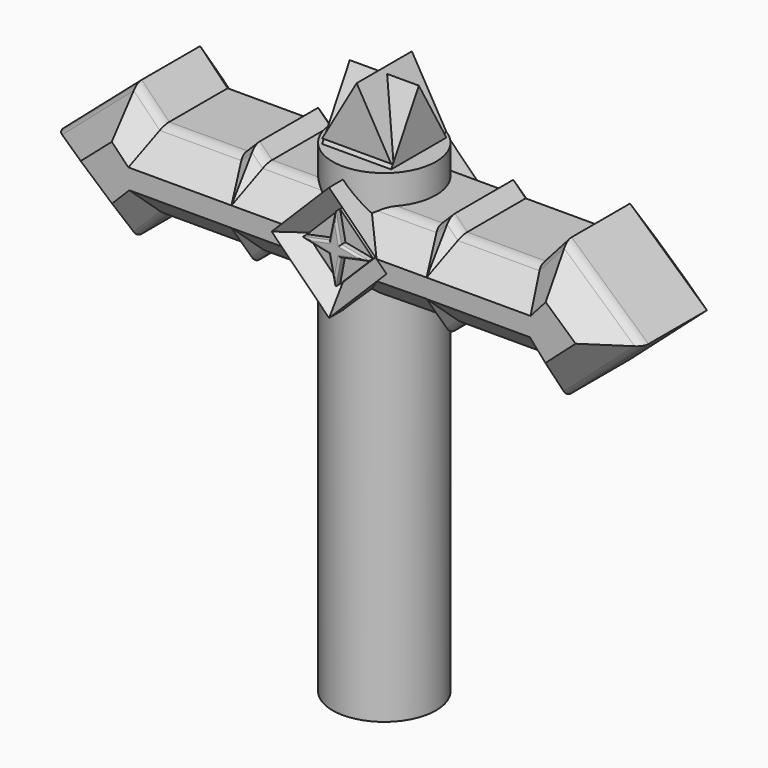
from build123d import *

# Parameters (mm, degrees)
F1_DEPTH  = 25.4
F2_DEPTH  = 25.4
F3_SIZE   = 6.34999
F4_DEPTH  = 22.86
F5_DEPTH  = 20.32
F6_R      = 0.762
F7_SIZE   = 10.922
F10_R     = 19.05
F11_DEPTH = 152.4
F12_R     = 19.05
F13_DEPTH = 25.4
F14_R     = 5.08
F17_DEPTH = 12.7
F18_DEPTH = 12.7


# Not quite as in the source:
# - a fillet or chamfer is up to 0.001 mm smaller than in the source, because OpenCascade refuses the exact size


with BuildPart() as f1:
    # F0 (on Front) → F1 (new body)
    with BuildSketch(Plane.XZ):
        Polygon((-79.349612556, -24.9440319331), (-79.349612556, 0), (-108.0387504357, 0), align=None)
        Polygon((-108.0387504357, 0), (-79.349612556, 0), (-79.349612556, 24.9440319331), align=None)
        Polygon((-79.349612556, 0), (-69.1079095973, 0), (-69.2396351026, 14.5706034692), (-79.349612556, 24.9440319331), align=None)
        Polygon((-68.976184092, -14.5706034692), (-69.1079095973, 0), (-79.349612556, 0), (-79.349612556, -24.9440319331), align=None)
        Polygon((-40.4525237048, -14.5706034692), (-40.4525237048, 0), (-69.1079095973, 0), (-68.976184092, -14.5706034692), align=None)
        Polygon((-69.1079095973, 0), (-40.4525237048, 0), (-40.4525237048, 14.5706034692), (-69.2396351026, 14.5706034692), align=None)
        Polygon((-40.4525237048, 0), (-31.3568816876, 0), (-31.3568816876, 14.5706034692), (-35.9047026962, 19.1184244778), (-40.4525237048, 14.5706034692), align=None)
        Polygon((-31.3568816876, -14.5706034692), (-31.3568816876, 0), (-40.4525237048, 0), (-40.4525237048, -14.5706034692), (-35.9047026962, -19.1184244778), align=None)
    extrude(amount=F1_DEPTH)

    # F0 (on Front) → F2 (join)
    with BuildSketch(Plane.XZ):
        Polygon((-31.3568816876, 0), (-21.1349201239, 0), (-6.5643166548, 14.5706034692), (-31.3568816876, 14.5706034692), align=None)
        Polygon((-6.5643166548, -14.5706034692), (-21.1349201239, 0), (-31.3568816876, 0), (-31.3568816876, -14.5706034692), align=None)
        Polygon((-6.5643166548, 14.5706034692), (-21.1349201239, 0), (-6.5643166548, -14.5706034692), (0, -21.1349201239), (6.5643166548, -14.5706034692), (21.1349201239, 0), (6.5643166548, 14.5706034692), (0, 21.1349201239), align=None)
        Polygon((-12.1546640029, 0), (0, 12.1546640029), (12.1546640029, 0), (0, -12.1546640029), align=None, mode=Mode.SUBTRACT)
        Polygon((21.1349201239, 0), (6.5643166548, -14.5706034692), (31.3547166548, -14.2429622819), (31.3547166548, 0), align=None)
        Polygon((31.3547166548, 14.5706034692), (6.5643166548, 14.5706034692), (21.1349201239, 0), (31.3547166548, 0), align=None)
        Polygon((35.898726252, 19.1146130664), (31.3547166548, 14.5706034692), (31.3547166548, 0), (40.4427358493, 0), (40.4427358493, 14.5706034692), align=None)
        Polygon((40.4427358493, 14.5706034692), (40.4427358493, 0), (69.0966238814, 0), (69.2298472471, 14.5706034692), align=None)
        Polygon((31.3547166548, 0), (31.3547166548, -14.2429622819), (35.898726252, -18.7869718792), (40.4427358493, -14.2429622819), (40.4427358493, 0), align=None)
        Polygon((69.0966238814, 0), (40.4427358493, 0), (40.4427358493, -14.2429622819), (68.9663962365, -14.2429622819), align=None)
        Polygon((78.6986056686, 0), (69.0966238814, 0), (68.9663962365, -14.2429622819), (78.6986056686, -25.2202176658), (78.7764995039, 0), align=None)
        Polygon((69.2298472471, 14.5706034692), (69.0966238814, 0), (78.6986056686, 0), (78.7764995039, 0), (78.8549345602, 25.3954524944), align=None)
        Polygon((107.1452571806, 0), (78.8549345602, 25.3954524944), (78.7764995039, 0), align=None)
        Polygon((78.7764995039, 0), (78.6986056686, -25.2202176658), (107.1452571806, 0), align=None)
    extrude(amount=F2_DEPTH)

    # F3 (size 6.35 in the source; OpenCascade refuses exactly that, so slightly less here)
    f3_edges = [f1.edges().sort_by_distance(p)[0] for p in [
        (-6.077332, -25.4, 6.077332),
        (6.077332, -25.4, 6.077332),
        (6.077332, -25.4, -6.077332),
        (-6.077332, -25.4, -6.077332),
    ]]
    chamfer(f3_edges, length=F3_SIZE)

    # F7
    f7_edges = [f1.edges().sort_by_distance(p)[0] for p in [
        (74.042391, -25.4, 19.983028),
        (93.000096, -25.4, 12.697726),
        (92.921931, -25.4, -12.610109),
        (73.832501, -25.4, -19.73159),
        (54.704566, -25.4, -14.242962),
        (54.836292, -25.4, 14.570603),
        (38.170731, -25.4, -16.514967),
        (33.626721, -25.4, -16.514967),
        (38.170731, -25.4, 16.842608),
        (33.626721, -25.4, 16.842608),
        (18.959517, -25.4, -14.406783),
        (18.959517, -25.4, 14.570603),
        (-18.960599, -25.4, -14.570603),
        (-33.630792, -25.4, -16.844514),
        (-54.714354, -25.4, -14.570603),
        (-74.162898, -25.4, -19.757318),
        (-93.694181, -25.4, -12.472016),
        (-38.178613, -25.4, -16.844514),
        (-18.960599, -25.4, 14.570603),
        (-33.630792, -25.4, 16.844514),
        (-38.178613, -25.4, 16.844514),
        (-54.846079, -25.4, 14.570603),
        (-74.294624, -25.4, 19.757318),
        (-93.694181, -25.4, 12.472016),
    ]]
    chamfer(f7_edges, length=F7_SIZE)

    # F8: F1 across plane


with BuildPart() as f4:
    # F0 (on Front) → F4 (new body)
    with BuildSketch(Plane.XZ):
        Polygon((1.9762939773, 2.0008223965), (0, 12.1546640029), (-2.1093236282, 2.0698737353), (-12.1546640029, 0), (-2.1093236282, -2.1010723321), (0, -12.1546640029), (1.9762939773, -2.1010723321), (12.1546640029, 0), align=None)
    extrude(amount=F4_DEPTH)

    # F6
    f6_edges = [f4.edges().sort_by_distance(p)[0] for p in [
        (7.065479, -22.86, 1.000411),
        (7.065479, -22.86, -1.050536),
        (0.988147, -22.86, -7.127868),
        (-1.054662, -22.86, -7.127868),
        (-7.131994, -22.86, -1.050536),
        (-7.131994, -22.86, 1.034937),
        (-1.054662, -22.86, 7.112269),
        (0.988147, -22.86, 7.077743),
    ]]
    fillet(f6_edges, radius=F6_R)


with BuildPart() as f5:
    # F0 (on Front) → F5 (new body)
    with BuildSketch(Plane.XZ):
        Polygon((12.1546640029, 0), (0, 12.1546640029), (1.9762939773, 2.0008223965), align=None)
    extrude(amount=F5_DEPTH)


with BuildPart() as f5b:
    # F0 (on Front) → F5, piece 2 (new body)
    with BuildSketch(Plane.XZ):
        Polygon((0, -12.1546640029), (12.1546640029, 0), (1.9762939773, -2.1010723321), align=None)
    extrude(amount=F5_DEPTH)


with BuildPart() as f5c:
    # F0 (on Front) → F5, piece 3 (new body)
    with BuildSketch(Plane.XZ):
        Polygon((-2.1093236282, -2.1010723321), (-12.1546640029, 0), (0, -12.1546640029), align=None)
    extrude(amount=F5_DEPTH)


with BuildPart() as f5d:
    # F0 (on Front) → F5, piece 4 (new body)
    with BuildSketch(Plane.XZ):
        Polygon((-2.1093236282, 2.0698737353), (0, 12.1546640029), (-12.1546640029, 0), align=None)
    extrude(amount=F5_DEPTH)


with BuildPart() as f1_1:
    add(f1.part)
    add(f1.part.mirror(Plane.XZ))

    # F14
    f14_edges = [f1_1.edges().sort_by_distance(p)[0] for p in [
        (93.000096, -14.478, 12.697726),
        (92.921931, -14.478, -12.610109),
        (74.042391, -14.478, 19.983028),
        (54.836292, -14.478, 14.570603),
        (54.704566, -14.478, -14.242962),
        (73.832501, -14.478, -19.73159),
        (18.959517, -14.478, -14.406783),
        (18.959517, -14.478, 14.570603),
        (33.626721, -14.478, -16.514967),
        (38.170731, -14.478, 16.842608),
        (-18.960599, -14.478, -14.570603),
        (-18.960599, -14.478, 14.570603),
        (-38.178613, -14.478, 16.844514),
        (-33.630792, -14.478, -16.844514),
        (-54.714354, -14.478, -14.570603),
        (-54.846079, -14.478, 14.570603),
        (-74.294624, -14.478, 19.757318),
        (-74.162898, -14.478, -19.757318),
        (-93.694181, -14.478, -12.472016),
        (-93.694181, -14.478, 12.472016),
        (-38.178613, -14.478, -16.844514),
        (-33.630792, -14.478, 16.844514),
        (33.626721, -14.478, 16.842608),
        (38.170731, -14.478, -16.514967),
    ]]
    fillet(f14_edges, radius=F14_R)


with BuildPart() as f9_1:
    # F9: instance of F4
    add(f4.part.mirror(Plane.XZ))


with BuildPart() as f9_2:
    # F9: instance of F5
    add(f5.part.mirror(Plane.XZ))


with BuildPart() as f9_3:
    # F9: instance of F5d
    add(f5d.part.mirror(Plane.XZ))


with BuildPart() as f9_4:
    # F9: instance of F5c
    add(f5c.part.mirror(Plane.XZ))


with BuildPart() as f9_5:
    # F9: instance of F5b
    add(f5b.part.mirror(Plane.XZ))


with BuildPart() as f11:
    # F10 (on Top) → F11 (new body)
    with BuildSketch(Plane.XY):
        Circle(F10_R)
    extrude(amount=-F11_DEPTH)


with BuildPart() as f13:
    # F12 (on Top) → F13 (new body)
    with BuildSketch(Plane.XY):
        Circle(F12_R)
    extrude(amount=F13_DEPTH)


with BuildPart() as f17:
    # F15 (on Front) → F17 (new body, symmetric)
    with BuildSketch(Plane.XZ):
        Polygon((12.7, 27.784103201), (0, 49.7811484571), (-12.7, 27.784103201), align=None)
    extrude(amount=F17_DEPTH, both=True)

    # F16 (on Right) → F18 (join, symmetric)
    with BuildSketch(Plane.YZ):
        Polygon((12.7, 25.9630926441), (0, 47.9601379003), (-12.7, 25.9630926441), align=None)
    extrude(amount=F18_DEPTH, both=True)


solid = Compound([f4.part, f5.part, f5b.part, f5c.part, f5d.part, f1_1.part, f9_1.part, f9_2.part, f9_3.part, f9_4.part, f9_5.part, f11.part, f13.part, f17.part])
